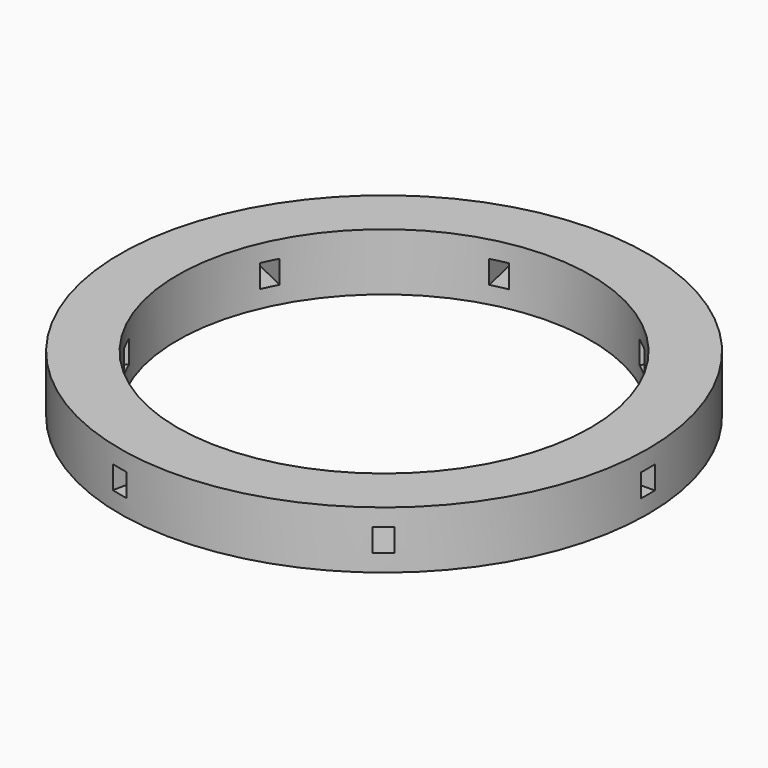
from build123d import *

# Parameters (mm, degrees)
F0_R            = 23
F0_R_2          = 18
F1_DEPTH        = 5
F2_W            = 1.5
F2_H            = 2
F3_DEPTH        = 23.001
F3_COPIES_COUNT = 7


# Not quite as in the source:
# - a pattern or mirror of a feature is missing from the dataset's text; its kind, count and spacing are read off the source's solid


with BuildPart() as f1:
    # F0 (on Top) → F1 (new body)
    with BuildSketch(Plane.XY):
        Circle(F0_R)
        Circle(F0_R_2, mode=Mode.SUBTRACT)
    extrude(amount=F1_DEPTH)

    # F2 (on Right) → F3 (cut, through all)
    with BuildSketch(Plane.YZ):
        with Locations((0, 2.5)):
            Rectangle(F2_W, F2_H)
    f3 = extrude(amount=F3_DEPTH, mode=Mode.SUBTRACT)

    # F3_copies: F3 ×7 about axis
    f3_copies_axis = Axis((0, 0, 0), (0, 0, 1))
    for i in range(1, F3_COPIES_COUNT):
        add(f3.rotate(f3_copies_axis, i * 360 / F3_COPIES_COUNT), mode=Mode.SUBTRACT)


solid = f1.part
